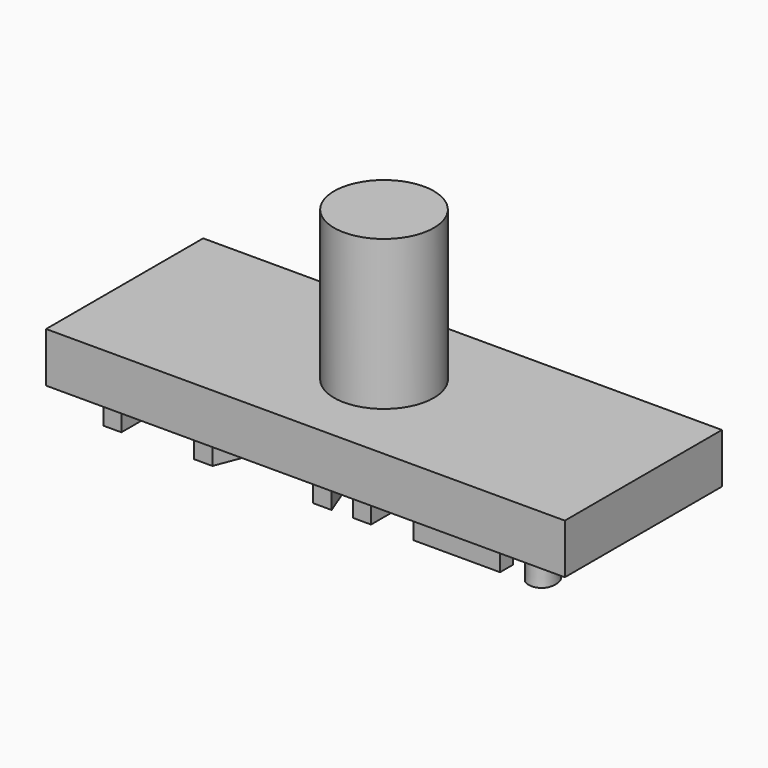
from build123d import *

# Parameters (mm, degrees)
F0_W         = 52
F0_H         = 19.684583747
F0_W_2       = 1.8074032052
F0_H_2       = 15.5518366189
F0_TEXT_SIZE = 21.784144093
F1_DEPTH     = 5
F2_DEPTH     = 3
F3_R         = 5
F4_DEPTH     = 15


# Not quite as in the source:
# - Text() gives the source's letters only with a copy of the font that has no kerning and outlines rounded to 1/6400 em; it was checked with that copy


with BuildPart() as f1:
    # F0 (on Top) → F1 (new body)
    with BuildSketch(Plane.XY):
        Rectangle(F0_W, F0_H)
        Polygon((-20.0550276557, -1.1947241526), (-20.0550276557, -7.8422918735), (-21.8624308609, -7.8422918735), (-21.8624308609, 7.7095447454), (-13.1930222663, 7.7095447454), (-13.1930222663, 6.1029641186), (-20.0550276557, 6.1029641186), (-20.0550276557, 0.4118564743), (-13.6082825131, 0.4118564743), (-13.6082825131, -1.1947241526), align=None, mode=Mode.SUBTRACT)
        Polygon((1.0279392994, -7.8422918735), (-0.8441355836, -7.8422918735), (-2.7808821444, -2.8966104099), (-9.0131896185, -2.8966104099), (-10.9261097717, -7.8422918735), (-12.7573393845, -7.8422918735), (-6.6101262232, 7.7742164232), (-5.0886399092, 7.7742164232), align=None, mode=Mode.SUBTRACT)
        with BuildLine():
            add(Edge.make_bspline(
                [(20.3868954758, -7.8167635796), (20.024393703, -7.481491987), (20.024393703, -6.7156431712)],
                knots=[0, 0, 0, 1, 1, 1], degree=2))
            add(Edge.make_bspline(
                [(20.024393703, -6.7156431712), (20.024393703, -5.2690398525), (21.300808396, -5.2690398525)],
                knots=[0, 0, 0, 1, 1, 1], degree=2))
            add(Edge.make_bspline(
                [(21.300808396, -5.2690398525), (21.9168912211, -5.2690398525), (22.2521628138, -5.6400510566)],
                knots=[0, 0, 0, 1, 1, 1], degree=2))
            add(Edge.make_bspline(
                [(22.2521628138, -5.6400510566), (22.5874344065, -6.0110622607), (22.5874344065, -6.7156431712)],
                knots=[0, 0, 0, 1, 1, 1], degree=2))
            add(Edge.make_bspline(
                [(22.5874344065, -6.7156431712), (22.5874344065, -7.3963976741), (22.247057155, -7.7742164232)],
                knots=[0, 0, 0, 1, 1, 1], degree=2))
            add(Edge.make_bspline(
                [(22.247057155, -7.7742164232), (21.9066799036, -8.1520351723), (21.300808396, -8.1520351723)],
                knots=[0, 0, 0, 1, 1, 1], degree=2))
            add(Edge.make_bspline(
                [(21.300808396, -8.1520351723), (20.7493972486, -8.1520351723), (20.3868954758, -7.8167635796)],
                knots=[0, 0, 0, 1, 1, 1], degree=2))
        make_face(mode=Mode.SUBTRACT)
        with Locations((4.0692100411, -0.066373564)):
            Rectangle(F0_W_2, F0_H_2, mode=Mode.SUBTRACT)
        Polygon((17.907247199, -7.8422918735), (9.2378386045, -7.8422918735), (9.2378386045, 7.7095447454), (11.0452418097, 7.7095447454), (11.0452418097, -6.205077294), (17.907247199, -6.205077294), align=None, mode=Mode.SUBTRACT)
        Polygon((22.4172457807, 7.7095447454), (21.8760459509, -3.5569422777), (20.7596085662, -3.5569422777), (20.2150049638, 7.7095447454), align=None, mode=Mode.SUBTRACT)
        with BuildLine():
            Line((-8.3732803858, -1.2696071479), (-3.3425046093, -1.2696071479))
            Line((-3.3425046093, -1.2696071479), (-5.153311587, 3.5501347327))
            add(Edge.make_bspline(
                [(-5.153311587, 3.5501347327), (-5.503900156, 4.4657495391), (-5.8749113601, 5.7932208197)],
                knots=[0, 0, 0, 1, 1, 1], degree=2))
            add(Edge.make_bspline(
                [(-5.8749113601, 5.7932208197), (-6.1097716636, 4.7720890654), (-6.5454545455, 3.5501347327)],
                knots=[0, 0, 0, 1, 1, 1], degree=2))
            Line((-6.5454545455, 3.5501347327), (-8.3732803858, -1.2696071479))
        make_face()
        with Locations((-24, -7.8422918735)):
            Text('FAIL!', F0_TEXT_SIZE, font='Open Sans', text_align=(TextAlign.LEFT, TextAlign.BOTTOM))
    extrude(amount=F1_DEPTH)

    # F0 (on Top) → F2 (join)
    with BuildSketch(Plane.XY):
        with Locations((-24, -7.8422918735)):
            Text('FAIL!', F0_TEXT_SIZE, font='Open Sans', text_align=(TextAlign.LEFT, TextAlign.BOTTOM))
    extrude(amount=-F2_DEPTH)

    # F3 (on face) → F4 (join)
    with BuildSketch(Plane.XY.offset(5)):
        Circle(F3_R)
    extrude(amount=F4_DEPTH)


solid = f1.part
